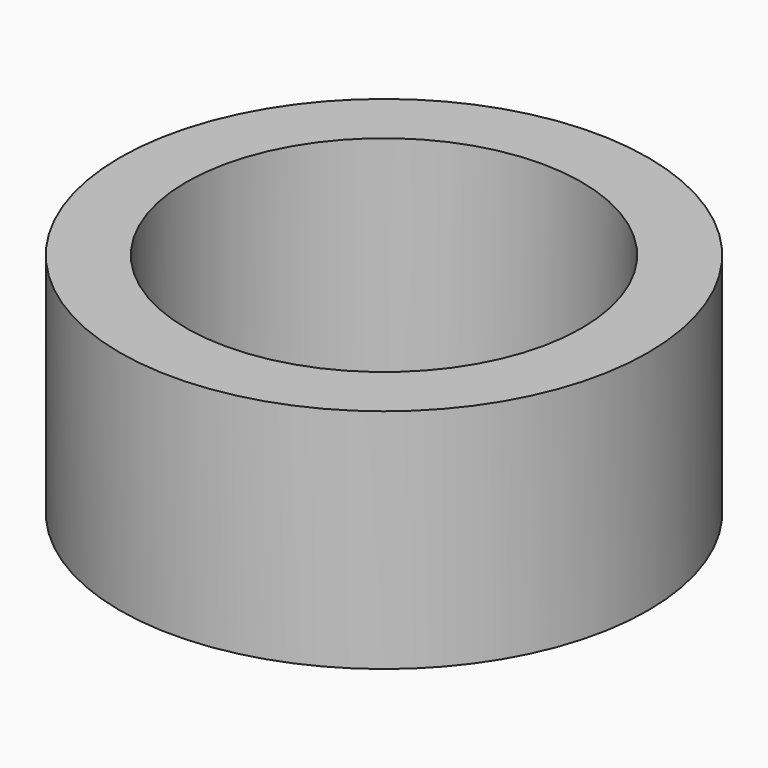
from build123d import *

# Parameters (mm, degrees)
F0_R     = 59.1258488549
F0_R_2   = 44.2629725155
F1_DEPTH = 50.8


# Not quite as in the source:
# - a feature names something its author has since deleted; it is built from what else it names


with BuildPart() as f1:
    # F0 (on Top) → F1 (new body)
    with BuildSketch(Plane.XY):
        Circle(F0_R)
        Circle(F0_R_2, mode=Mode.SUBTRACT)
    extrude(amount=F1_DEPTH)


solid = f1.part
